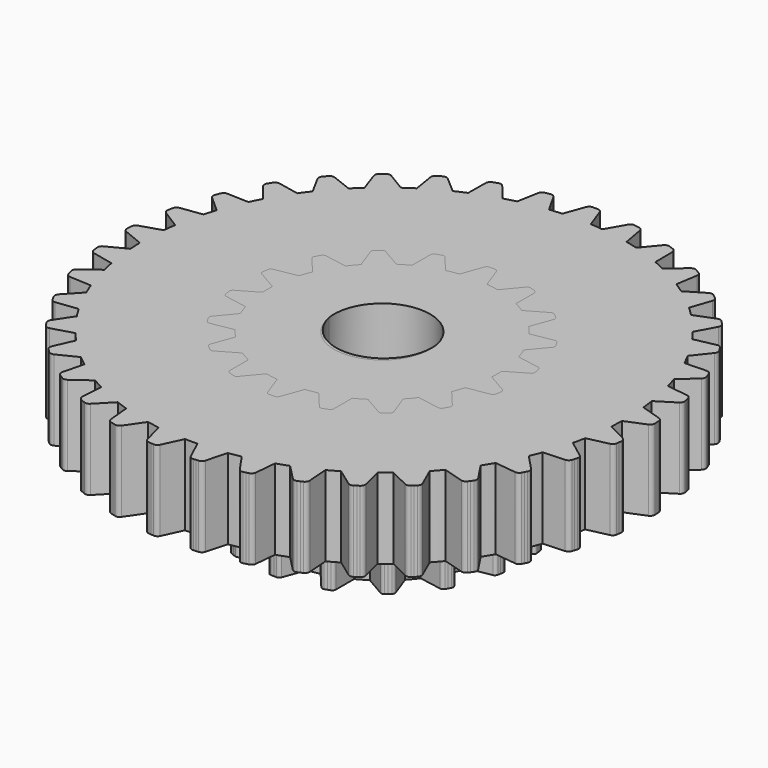
from build123d import *

# Parameters (mm, degrees)
F0_R      = 4.175
F1_DEPTH  = 7
F3_R      = 4.175
F4_DEPTH  = 7
F2_R      = 4.175
F5_DEPTH  = 7
F6_W      = 6
F6_H      = 6
F7_DEPTH  = 3.3
F8_R      = 1.65
F8_R_2    = 0.5
F9_DEPTH  = 0.2
F10_R     = 1.65
F11_DEPTH = 0.7


with BuildPart() as f1:
    # F0 (on Top) → F1 (new body)
    with BuildSketch(Plane.XY):
        with BuildLine():
            ThreePointArc((9.9853543406, -0.5410163509), (9.9963379146, -0.2706072741), (10, 0))
            ThreePointArc((10, 0), (9.9963379146, 0.2706072741), (9.9853543406, 0.5410163509))
            ThreePointArc((9.9853543406, 0.5410163509), (9.8480775301, 1.7364817767), (9.5682022797, 2.9068032501))
            ThreePointArc((9.5682022797, 2.9068032501), (9.3969262079, 3.4202014333), (9.1981253, 3.9235813954))
            ThreePointArc((9.1981253, 3.9235813954), (8.6602540378, 5), (7.9969838122, 6.0040194793))
            ThreePointArc((7.9969838122, 6.0040194793), (7.6604444312, 6.4278760969), (7.3014665983, 6.8329046177))
            ThreePointArc((7.3014665983, 6.8329046177), (6.4278760969, 7.6604444312), (5.461211074, 8.3770623494))
            ThreePointArc((5.461211074, 8.3770623494), (5, 8.6602540378), (4.5241432666, 8.9180787002))
            ThreePointArc((4.5241432666, 8.9180787002), (3.4202014333, 9.3969262079), (2.2667356814, 9.7397078678))
            ThreePointArc((2.2667356814, 9.7397078678), (1.7364817767, 9.8480775301), (1.2011414878, 9.9276008746))
            ThreePointArc((1.2011414878, 9.9276008746), (0.601660724, 9.9818838088), (0, 10))
            ThreePointArc((0, 10), (-0.601660724, 9.9818838088), (-1.2011414878, 9.9276008746))
            ThreePointArc((-1.2011414878, 9.9276008746), (-1.7364817767, 9.8480775301), (-2.2667356814, 9.7397078678))
            ThreePointArc((-2.2667356814, 9.7397078678), (-3.4202014333, 9.3969262079), (-4.5241432666, 8.9180787002))
            ThreePointArc((-4.5241432666, 8.9180787002), (-5, 8.6602540378), (-5.461211074, 8.3770623494))
            ThreePointArc((-5.461211074, 8.3770623494), (-6.4278760969, 7.6604444312), (-7.3014665983, 6.8329046177))
            ThreePointArc((-7.3014665983, 6.8329046177), (-7.6604444312, 6.4278760969), (-7.9969838122, 6.0040194793))
            ThreePointArc((-7.9969838122, 6.0040194793), (-8.6602540378, 5), (-9.1981253, 3.9235813954))
            ThreePointArc((-9.1981253, 3.9235813954), (-9.3969262079, 3.4202014333), (-9.5682022797, 2.9068032501))
            ThreePointArc((-9.5682022797, 2.9068032501), (-9.8480775301, 1.7364817767), (-9.9853543406, 0.5410163509))
            ThreePointArc((-9.9853543406, 0.5410163509), (-10, 0), (-9.9853543406, -0.5410163509))
            ThreePointArc((-9.9853543406, -0.5410163509), (-9.8480775301, -1.7364817767), (-9.5682022797, -2.9068032501))
            ThreePointArc((-9.5682022797, -2.9068032501), (-9.3969262079, -3.4202014333), (-9.1981253, -3.9235813954))
            ThreePointArc((-9.1981253, -3.9235813954), (-8.6602540378, -5), (-7.9969838122, -6.0040194793))
            ThreePointArc((-7.9969838122, -6.0040194793), (-7.6604444312, -6.4278760969), (-7.3014665983, -6.8329046177))
            ThreePointArc((-7.3014665983, -6.8329046177), (-6.4278760969, -7.6604444312), (-5.461211074, -8.3770623494))
            ThreePointArc((-5.461211074, -8.3770623494), (-5, -8.6602540378), (-4.5241432666, -8.9180787002))
            ThreePointArc((-4.5241432666, -8.9180787002), (-3.4202014333, -9.3969262079), (-2.2667356814, -9.7397078678))
            ThreePointArc((-2.2667356814, -9.7397078678), (-1.7364817767, -9.8480775301), (-1.2011414878, -9.9276008746))
            ThreePointArc((-1.2011414878, -9.9276008746), (0, -10), (1.2011414878, -9.9276008746))
            ThreePointArc((1.2011414878, -9.9276008746), (1.7364817767, -9.8480775301), (2.2667356814, -9.7397078678))
            ThreePointArc((2.2667356814, -9.7397078678), (3.4202014333, -9.3969262079), (4.5241432666, -8.9180787002))
            ThreePointArc((4.5241432666, -8.9180787002), (5, -8.6602540378), (5.461211074, -8.3770623494))
            ThreePointArc((5.461211074, -8.3770623494), (6.4278760969, -7.6604444312), (7.3014665983, -6.8329046177))
            ThreePointArc((7.3014665983, -6.8329046177), (7.6604444312, -6.4278760969), (7.9969838122, -6.0040194793))
            ThreePointArc((7.9969838122, -6.0040194793), (8.6602540378, -5), (9.1981253, -3.9235813954))
            ThreePointArc((9.1981253, -3.9235813954), (9.3969262079, -3.4202014333), (9.5682022797, -2.9068032501))
            ThreePointArc((9.5682022797, -2.9068032501), (9.8480775301, -1.7364817767), (9.9853543406, -0.5410163509))
        make_face()
        Circle(F0_R, mode=Mode.SUBTRACT)
        with BuildLine():
            ThreePointArc((9.5682022797, 2.9068032501), (9.8480775301, 1.7364817767), (9.9853543406, 0.5410163509))
            Line((9.9853543406, 0.5410163509), (11.7091989464, 1.5362784981))
            ThreePointArc((11.7091989464, 1.5362784981), (11.8298906667, 1.6667571102), (11.8555661055, 1.8426318708))
            Line((11.8555661055, 1.8426318708), (11.8176930361, 2.083778132))
            Line((11.8176930361, 2.083778132), (11.7708052012, 2.3233348468))
            ThreePointArc((11.7708052012, 2.3233348468), (11.68652547, 2.4798215442), (11.5284860374, 2.5611523338))
            Line((11.5284860374, 2.5611523338), (9.5682022797, 2.9068032501))
        make_face()
        with BuildLine():
            Line((11.7091989464, -1.5362784981), (9.9853543406, -0.5410163509))
            ThreePointArc((9.9853543406, -0.5410163509), (9.8480775301, -1.7364817767), (9.5682022797, -2.9068032501))
            Line((9.5682022797, -2.9068032501), (11.5284860374, -2.5611523338))
            ThreePointArc((11.5284860374, -2.5611523338), (11.68652547, -2.4798215442), (11.7708052012, -2.3233348468))
            Line((11.7708052012, -2.3233348468), (11.8176930361, -2.083778132))
            Line((11.8176930361, -2.083778132), (11.8555661055, -1.8426318708))
            ThreePointArc((11.8555661055, -1.8426318708), (11.8298906667, -1.6667571102), (11.7091989464, -1.5362784981))
        make_face()
        with BuildLine():
            ThreePointArc((7.9969838122, 6.0040194793), (8.6602540378, 5), (9.1981253, 3.9235813954))
            Line((9.1981253, 3.9235813954), (10.4776096532, 5.44841147))
            ThreePointArc((10.4776096532, 5.44841147), (10.5463964585, 5.6123002585), (10.5103707681, 5.7863499905))
            Line((10.5103707681, 5.7863499905), (10.3923048454, 6))
            Line((10.3923048454, 6), (10.266311471, 6.2090730931))
            ThreePointArc((10.266311471, 6.2090730931), (10.1335928268, 6.3272971222), (9.9572675699, 6.3496703956))
            Line((9.9572675699, 6.3496703956), (7.9969838122, 6.0040194793))
        make_face()
        with BuildLine():
            Line((10.4776096532, -5.44841147), (9.1981253, -3.9235813954))
            ThreePointArc((9.1981253, -3.9235813954), (8.6602540378, -5), (7.9969838122, -6.0040194793))
            Line((7.9969838122, -6.0040194793), (9.9572675699, -6.3496703956))
            ThreePointArc((9.9572675699, -6.3496703956), (10.1335928268, -6.3272971222), (10.266311471, -6.2090730931))
            Line((10.266311471, -6.2090730931), (10.3923048454, -6))
            Line((10.3923048454, -6), (10.5103707681, -5.7863499905))
            ThreePointArc((10.5103707681, -5.7863499905), (10.5463964585, -5.6123002585), (10.4776096532, -5.44841147))
        make_face()
        with BuildLine():
            ThreePointArc((5.461211074, 8.3770623494), (6.4278760969, 7.6604444312), (7.3014665983, 6.8329046177))
            Line((7.3014665983, 6.8329046177), (7.9822660027, 8.7033856086))
            ThreePointArc((7.9822660027, 8.7033856086), (7.9908511891, 8.8809171668), (7.8974695994, 9.0321489038))
            Line((7.8974695994, 9.0321489038), (7.7134513162, 9.1925333174))
            Line((7.7134513162, 9.1925333174), (7.5235490627, 9.3459054882))
            ThreePointArc((7.5235490627, 9.3459054882), (7.3583993328, 9.4116072863), (7.1850556798, 9.3723244965))
            Line((7.1850556798, 9.3723244965), (5.461211074, 8.3770623494))
        make_face()
        with BuildLine():
            Line((7.9822660027, -8.7033856086), (7.3014665983, -6.8329046177))
            ThreePointArc((7.3014665983, -6.8329046177), (6.4278760969, -7.6604444312), (5.461211074, -8.3770623494))
            Line((5.461211074, -8.3770623494), (7.1850556798, -9.3723244965))
            ThreePointArc((7.1850556798, -9.3723244965), (7.3583993328, -9.4116072863), (7.5235490627, -9.3459054882))
            Line((7.5235490627, -9.3459054882), (7.7134513162, -9.1925333174))
            Line((7.7134513162, -9.1925333174), (7.8974695994, -9.0321489038))
            ThreePointArc((7.8974695994, -9.0321489038), (7.9908511891, -8.8809171668), (7.9822660027, -8.7033856086))
        make_face()
        with BuildLine():
            ThreePointArc((2.2667356814, 9.7397078678), (3.4202014333, 9.3969262079), (4.5241432666, 8.9180787002))
            Line((4.5241432666, 8.9180787002), (4.5241432666, 10.9086029946))
            ThreePointArc((4.5241432666, 10.9086029946), (4.471491334, 11.0783643965), (4.3320170428, 11.1885373591))
            Line((4.3320170428, 11.1885373591), (4.1042417199, 11.2763114494))
            Line((4.1042417199, 11.2763114494), (3.8733356018, 11.3554837506))
            ThreePointArc((3.8733356018, 11.3554837506), (3.6956742808, 11.3607387111), (3.5462200347, 11.2645379424))
            Line((3.5462200347, 11.2645379424), (2.2667356814, 9.7397078678))
        make_face()
        with BuildLine():
            Line((4.5241432666, -10.9086029946), (4.5241432666, -8.9180787002))
            ThreePointArc((4.5241432666, -8.9180787002), (3.4202014333, -9.3969262079), (2.2667356814, -9.7397078678))
            Line((2.2667356814, -9.7397078678), (3.5462200347, -11.2645379424))
            ThreePointArc((3.5462200347, -11.2645379424), (3.6956742808, -11.3607387111), (3.8733356018, -11.3554837506))
            Line((3.8733356018, -11.3554837506), (4.1042417199, -11.2763114494))
            Line((4.1042417199, -11.2763114494), (4.3320170428, -11.1885373591))
            ThreePointArc((4.3320170428, -11.1885373591), (4.471491334, -11.0783643965), (4.5241432666, -10.9086029946))
        make_face()
        with BuildLine():
            ThreePointArc((0, 10), (0.601660724, 9.9818838088), (1.2011414878, 9.9276008746))
            Line((1.2011414878, 9.9276008746), (0.5203420833, 11.7980818656))
            ThreePointArc((0.5203420833, 11.7980818656), (0.4128036317, 11.9395973807), (0.2440592971, 11.9954230836))
            Line((0.2440592971, 11.9954230836), (0, 12))
            Line((0, 12), (0, 10))
        make_face()
        with BuildLine():
            Line((0.5203420833, -11.7980818656), (1.2011414878, -9.9276008746))
            ThreePointArc((1.2011414878, -9.9276008746), (0, -10), (-1.2011414878, -9.9276008746))
            Line((-1.2011414878, -9.9276008746), (-0.5203420833, -11.7980818656))
            ThreePointArc((-0.5203420833, -11.7980818656), (-0.4128036317, -11.9395973807), (-0.2440592971, -11.9954230836))
            Line((-0.2440592971, -11.9954230836), (0, -12))
            Line((0, -12), (0.2440592971, -11.9954230836))
            ThreePointArc((0.2440592971, -11.9954230836), (0.4128036317, -11.9395973807), (0.5203420833, -11.7980818656))
        make_face()
        with BuildLine():
            ThreePointArc((-1.2011414878, 9.9276008746), (-0.601660724, 9.9818838088), (0, 10))
            Line((0, 10), (0, 12))
            Line((0, 12), (-0.2440592971, 11.9954230836))
            ThreePointArc((-0.2440592971, 11.9954230836), (-0.4128036317, 11.9395973807), (-0.5203420833, 11.7980818656))
            Line((-0.5203420833, 11.7980818656), (-1.2011414878, 9.9276008746))
        make_face()
        with BuildLine():
            Line((-3.5462200347, -11.2645379424), (-2.2667356814, -9.7397078678))
            ThreePointArc((-2.2667356814, -9.7397078678), (-3.4202014333, -9.3969262079), (-4.5241432666, -8.9180787002))
            Line((-4.5241432666, -8.9180787002), (-4.5241432666, -10.9086029946))
            ThreePointArc((-4.5241432666, -10.9086029946), (-4.471491334, -11.0783643965), (-4.3320170428, -11.1885373591))
            Line((-4.3320170428, -11.1885373591), (-4.1042417199, -11.2763114494))
            Line((-4.1042417199, -11.2763114494), (-3.8733356018, -11.3554837506))
            ThreePointArc((-3.8733356018, -11.3554837506), (-3.6956742808, -11.3607387111), (-3.5462200347, -11.2645379424))
        make_face()
        with BuildLine():
            ThreePointArc((-4.5241432666, 8.9180787002), (-3.4202014333, 9.3969262079), (-2.2667356814, 9.7397078678))
            Line((-2.2667356814, 9.7397078678), (-3.5462200347, 11.2645379424))
            ThreePointArc((-3.5462200347, 11.2645379424), (-3.6956742808, 11.3607387111), (-3.8733356018, 11.3554837506))
            Line((-3.8733356018, 11.3554837506), (-4.1042417199, 11.2763114494))
            Line((-4.1042417199, 11.2763114494), (-4.3320170428, 11.1885373591))
            ThreePointArc((-4.3320170428, 11.1885373591), (-4.471491334, 11.0783643965), (-4.5241432666, 10.9086029946))
            Line((-4.5241432666, 10.9086029946), (-4.5241432666, 8.9180787002))
        make_face()
        with BuildLine():
            Line((-7.1850556798, -9.3723244965), (-5.461211074, -8.3770623494))
            ThreePointArc((-5.461211074, -8.3770623494), (-6.4278760969, -7.6604444312), (-7.3014665983, -6.8329046177))
            Line((-7.3014665983, -6.8329046177), (-7.9822660027, -8.7033856086))
            ThreePointArc((-7.9822660027, -8.7033856086), (-7.9908511891, -8.8809171668), (-7.8974695994, -9.0321489038))
            Line((-7.8974695994, -9.0321489038), (-7.7134513162, -9.1925333174))
            Line((-7.7134513162, -9.1925333174), (-7.5235490627, -9.3459054882))
            ThreePointArc((-7.5235490627, -9.3459054882), (-7.3583993328, -9.4116072863), (-7.1850556798, -9.3723244965))
        make_face()
        with BuildLine():
            ThreePointArc((-7.3014665983, 6.8329046177), (-6.4278760969, 7.6604444312), (-5.461211074, 8.3770623494))
            Line((-5.461211074, 8.3770623494), (-7.1850556798, 9.3723244965))
            ThreePointArc((-7.1850556798, 9.3723244965), (-7.3583993328, 9.4116072863), (-7.5235490627, 9.3459054882))
            Line((-7.5235490627, 9.3459054882), (-7.7134513162, 9.1925333174))
            Line((-7.7134513162, 9.1925333174), (-7.8974695994, 9.0321489038))
            ThreePointArc((-7.8974695994, 9.0321489038), (-7.9908511891, 8.8809171668), (-7.9822660027, 8.7033856086))
            Line((-7.9822660027, 8.7033856086), (-7.3014665983, 6.8329046177))
        make_face()
        with BuildLine():
            Line((-9.9572675699, -6.3496703956), (-7.9969838122, -6.0040194793))
            ThreePointArc((-7.9969838122, -6.0040194793), (-8.6602540378, -5), (-9.1981253, -3.9235813954))
            Line((-9.1981253, -3.9235813954), (-10.4776096532, -5.44841147))
            ThreePointArc((-10.4776096532, -5.44841147), (-10.5463964585, -5.6123002585), (-10.5103707681, -5.7863499905))
            Line((-10.5103707681, -5.7863499905), (-10.3923048454, -6))
            Line((-10.3923048454, -6), (-10.266311471, -6.2090730931))
            ThreePointArc((-10.266311471, -6.2090730931), (-10.1335928268, -6.3272971222), (-9.9572675699, -6.3496703956))
        make_face()
        with BuildLine():
            ThreePointArc((-9.1981253, 3.9235813954), (-8.6602540378, 5), (-7.9969838122, 6.0040194793))
            Line((-7.9969838122, 6.0040194793), (-9.9572675699, 6.3496703956))
            ThreePointArc((-9.9572675699, 6.3496703956), (-10.1335928268, 6.3272971222), (-10.266311471, 6.2090730931))
            Line((-10.266311471, 6.2090730931), (-10.3923048454, 6))
            Line((-10.3923048454, 6), (-10.5103707681, 5.7863499905))
            ThreePointArc((-10.5103707681, 5.7863499905), (-10.5463964585, 5.6123002585), (-10.4776096532, 5.44841147))
            Line((-10.4776096532, 5.44841147), (-9.1981253, 3.9235813954))
        make_face()
        with BuildLine():
            Line((-11.5284860374, -2.5611523338), (-9.5682022797, -2.9068032501))
            ThreePointArc((-9.5682022797, -2.9068032501), (-9.8480775301, -1.7364817767), (-9.9853543406, -0.5410163509))
            Line((-9.9853543406, -0.5410163509), (-11.7091989464, -1.5362784981))
            ThreePointArc((-11.7091989464, -1.5362784981), (-11.8298906667, -1.6667571102), (-11.8555661055, -1.8426318708))
            Line((-11.8555661055, -1.8426318708), (-11.8176930361, -2.083778132))
            Line((-11.8176930361, -2.083778132), (-11.7708052012, -2.3233348468))
            ThreePointArc((-11.7708052012, -2.3233348468), (-11.68652547, -2.4798215442), (-11.5284860374, -2.5611523338))
        make_face()
        with BuildLine():
            ThreePointArc((-9.9853543406, 0.5410163509), (-9.8480775301, 1.7364817767), (-9.5682022797, 2.9068032501))
            Line((-9.5682022797, 2.9068032501), (-11.5284860374, 2.5611523338))
            ThreePointArc((-11.5284860374, 2.5611523338), (-11.68652547, 2.4798215442), (-11.7708052012, 2.3233348468))
            Line((-11.7708052012, 2.3233348468), (-11.8176930361, 2.083778132))
            Line((-11.8176930361, 2.083778132), (-11.8555661055, 1.8426318708))
            ThreePointArc((-11.8555661055, 1.8426318708), (-11.8298906667, 1.6667571102), (-11.7091989464, 1.5362784981))
            Line((-11.7091989464, 1.5362784981), (-9.9853543406, 0.5410163509))
        make_face()
    extrude(amount=F1_DEPTH)

    # F2 (on face) → F5 (join)
    with BuildSketch(Plane.XY.offset(7)):
        with BuildLine():
            ThreePointArc((20.9971088354, -0.3484545248), (20.9992771964, -0.1742332594), (21, 0))
            ThreePointArc((21, 0), (20.9729614688, 1.0653108598), (20.8919155021, 2.1278784395))
            ThreePointArc((20.8919155021, 2.1278784395), (20.8299091404, 2.6673742147), (20.75397364, 3.2050862938))
            ThreePointArc((20.75397364, 3.2050862938), (20.5286600179, 4.4242646699), (20.2317911147, 5.6280217032))
            ThreePointArc((20.2317911147, 5.6280217032), (20.0795014295, 6.1492781968), (19.9137844096, 6.6664226153))
            ThreePointArc((19.9137844096, 6.6664226153), (19.4856695732, 7.8299860334), (18.9896349328, 8.9662570294))
            ThreePointArc((18.9896349328, 8.9662570294), (18.7514430211, 9.4542786412), (18.5007118588, 9.9359780957))
            ThreePointArc((18.5007118588, 9.9359780957), (17.8821118924, 11.0104529547), (17.2011815283, 12.0465494658))
            ThreePointArc((17.2011815283, 12.0465494658), (16.8839397377, 12.4872967024), (16.5554075119, 12.9196935767))
            ThreePointArc((16.5554075119, 12.9196935767), (15.7641184103, 13.8741691912), (14.9178814493, 14.780284607))
            ThreePointArc((14.9178814493, 14.780284607), (14.5307162485, 15.161077973), (14.1338342332, 15.5317329963))
            ThreePointArc((14.1338342332, 15.5317329963), (13.1926199432, 16.3387508407), (12.2054210819, 17.0888178705))
            ThreePointArc((12.2054210819, 17.0888178705), (11.7594705089, 17.3987026341), (11.3056562771, 17.6969527361))
            ThreePointArc((11.3056562771, 17.6969527361), (10.2415938201, 18.3332963764), (9.1418329724, 18.9057369575))
            ThreePointArc((9.1418329724, 18.9057369575), (8.6499262131, 19.1357982982), (8.152235174, 19.3530633665))
            ThreePointArc((8.152235174, 19.3530633665), (6.9959356896, 19.8004263547), (5.8152509727, 20.1787724137))
            ThreePointArc((5.8152509727, 20.1787724137), (5.2915392891, 20.3223918856), (4.7642891078, 20.4524215998))
            ThreePointArc((4.7642891078, 20.4524215998), (3.5490172268, 20.6979341173), (2.3213747904, 20.871301327))
            ThreePointArc((2.3213747904, 20.871301327), (1.780924414, 20.9243472594), (1.2392831182, 20.9634009014))
            ThreePointArc((1.2392831182, 20.9634009014), (0, 21), (-1.2392831182, 20.9634009014))
            ThreePointArc((-1.2392831182, 20.9634009014), (-1.780924414, 20.9243472594), (-2.3213747904, 20.871301327))
            ThreePointArc((-2.3213747904, 20.871301327), (-3.5490172268, 20.6979341173), (-4.7642891078, 20.4524215998))
            ThreePointArc((-4.7642891078, 20.4524215998), (-5.2915392891, 20.3223918856), (-5.8152509727, 20.1787724137))
            ThreePointArc((-5.8152509727, 20.1787724137), (-6.9959356896, 19.8004263547), (-8.152235174, 19.3530633665))
            ThreePointArc((-8.152235174, 19.3530633665), (-8.6499262131, 19.1357982982), (-9.1418329724, 18.9057369575))
            ThreePointArc((-9.1418329724, 18.9057369575), (-10.2415938201, 18.3332963764), (-11.3056562771, 17.6969527361))
            ThreePointArc((-11.3056562771, 17.6969527361), (-11.7594705089, 17.3987026341), (-12.2054210819, 17.0888178705))
            ThreePointArc((-12.2054210819, 17.0888178705), (-13.1926199432, 16.3387508407), (-14.1338342332, 15.5317329963))
            ThreePointArc((-14.1338342332, 15.5317329963), (-14.5307162485, 15.161077973), (-14.9178814493, 14.780284607))
            ThreePointArc((-14.9178814493, 14.780284607), (-15.7641184103, 13.8741691912), (-16.5554075119, 12.9196935767))
            ThreePointArc((-16.5554075119, 12.9196935767), (-16.8839397377, 12.4872967024), (-17.2011815283, 12.0465494658))
            ThreePointArc((-17.2011815283, 12.0465494658), (-17.8821118924, 11.0104529547), (-18.5007118588, 9.9359780957))
            ThreePointArc((-18.5007118588, 9.9359780957), (-18.7514430211, 9.4542786412), (-18.9896349328, 8.9662570294))
            ThreePointArc((-18.9896349328, 8.9662570294), (-19.4856695732, 7.8299860334), (-19.9137844096, 6.6664226153))
            ThreePointArc((-19.9137844096, 6.6664226153), (-20.0795014295, 6.1492781968), (-20.2317911147, 5.6280217032))
            ThreePointArc((-20.2317911147, 5.6280217032), (-20.5286600179, 4.4242646699), (-20.75397364, 3.2050862938))
            ThreePointArc((-20.75397364, 3.2050862938), (-20.8299091404, 2.6673742147), (-20.8919155021, 2.1278784395))
            ThreePointArc((-20.8919155021, 2.1278784395), (-20.9810782903, 0.8912652671), (-20.9971088354, -0.3484545248))
            ThreePointArc((-20.9971088354, -0.3484545248), (-20.9810782903, -0.8912652671), (-20.9510175183, -1.4334800127))
            ThreePointArc((-20.9510175183, -1.4334800127), (-20.8299091404, -2.6673742147), (-20.6361954389, -3.8919709413))
            ThreePointArc((-20.6361954389, -3.8919709413), (-20.5286600179, -4.4242646699), (-20.407396906, -4.9535998548))
            ThreePointArc((-20.407396906, -4.9535998548), (-20.0795014295, -6.1492781968), (-19.6816162719, -7.3235224398))
            ThreePointArc((-19.6816162719, -7.3235224398), (-19.4856695732, -7.8299860334), (-19.2766926403, -8.3312136482))
            ThreePointArc((-19.2766926403, -8.3312136482), (-18.7514430211, -9.4542786412), (-18.1608328389, -10.5443895317))
            ThreePointArc((-18.1608328389, -10.5443895317), (-17.8821118924, -11.0104529547), (-17.5914330244, -11.4691535934))
            ThreePointArc((-17.5914330244, -11.4691535934), (-16.8839397377, -12.4872967024), (-16.1175953106, -13.4619137349))
            ThreePointArc((-16.1175953106, -13.4619137349), (-15.7641184103, -13.8741691912), (-15.4000999089, -14.2771468717))
            ThreePointArc((-15.4000999089, -14.2771468717), (-14.5307162485, -15.161077973), (-13.6106839104, -15.9921631899))
            ThreePointArc((-13.6106839104, -15.9921631899), (-13.1926199432, -16.3387508407), (-12.765733958, -16.6744126287))
            ThreePointArc((-12.765733958, -16.6744126287), (-11.7594705089, -17.3987026341), (-10.7122179149, -18.0623472268))
            ThreePointArc((-10.7122179149, -18.0623472268), (-10.2415938201, -18.3332963764), (-9.7641210837, -18.5919858935))
            ThreePointArc((-9.7641210837, -18.5919858935), (-8.6499262131, -19.1357982982), (-7.5055809138, -19.6129104201))
            ThreePointArc((-7.5055809138, -19.6129104201), (-6.9959356896, -19.8004263547), (-6.4816122232, -19.9747015744))
            ThreePointArc((-6.4816122232, -19.9747015744), (-5.2915392891, -20.3223918856), (-4.0830220152, -20.5992458897))
            ThreePointArc((-4.0830220152, -20.5992458897), (-3.5490172268, -20.6979341173), (-3.0126391801, -20.7827814589))
            ThreePointArc((-3.0126391801, -20.7827814589), (-1.780924414, -20.9243472594), (-0.5430020071, -20.99297856))
            ThreePointArc((-0.5430020071, -20.99297856), (0, -21), (0.5430020071, -20.99297856))
            ThreePointArc((0.5430020071, -20.99297856), (1.780924414, -20.9243472594), (3.0126391801, -20.7827814589))
            ThreePointArc((3.0126391801, -20.7827814589), (3.5490172268, -20.6979341173), (4.0830220152, -20.5992458897))
            ThreePointArc((4.0830220152, -20.5992458897), (5.2915392891, -20.3223918856), (6.4816122232, -19.9747015744))
            ThreePointArc((6.4816122232, -19.9747015744), (6.9959356896, -19.8004263547), (7.5055809138, -19.6129104201))
            ThreePointArc((7.5055809138, -19.6129104201), (8.6499262131, -19.1357982982), (9.7641210837, -18.5919858935))
            ThreePointArc((9.7641210837, -18.5919858935), (10.2415938201, -18.3332963764), (10.7122179149, -18.0623472268))
            ThreePointArc((10.7122179149, -18.0623472268), (11.7594705089, -17.3987026341), (12.765733958, -16.6744126287))
            ThreePointArc((12.765733958, -16.6744126287), (13.1926199432, -16.3387508407), (13.6106839104, -15.9921631899))
            ThreePointArc((13.6106839104, -15.9921631899), (14.5307162485, -15.161077973), (15.4000999089, -14.2771468717))
            ThreePointArc((15.4000999089, -14.2771468717), (15.7641184103, -13.8741691912), (16.1175953106, -13.4619137349))
            ThreePointArc((16.1175953106, -13.4619137349), (16.8839397377, -12.4872967024), (17.5914330244, -11.4691535934))
            ThreePointArc((17.5914330244, -11.4691535934), (17.8821118924, -11.0104529547), (18.1608328389, -10.5443895317))
            ThreePointArc((18.1608328389, -10.5443895317), (18.7514430211, -9.4542786412), (19.2766926403, -8.3312136482))
            ThreePointArc((19.2766926403, -8.3312136482), (19.4856695732, -7.8299860334), (19.6816162719, -7.3235224398))
            ThreePointArc((19.6816162719, -7.3235224398), (20.0795014295, -6.1492781968), (20.407396906, -4.9535998548))
            ThreePointArc((20.407396906, -4.9535998548), (20.5286600179, -4.4242646699), (20.6361954389, -3.8919709413))
            ThreePointArc((20.6361954389, -3.8919709413), (20.8299091404, -2.6673742147), (20.9510175183, -1.4334800127))
            ThreePointArc((20.9510175183, -1.4334800127), (20.9810782903, -0.8912652671), (20.9971088354, -0.3484545248))
        make_face()
        Circle(F2_R, mode=Mode.SUBTRACT)
        with BuildLine():
            ThreePointArc((20.8919155021, 2.1278784395), (20.9729614688, 1.0653108598), (21, 0))
            ThreePointArc((21, 0), (20.9992771964, -0.1742332594), (20.9971088354, -0.3484545248))
            Line((20.9971088354, -0.3484545248), (22.7391606338, 0.370721297))
            ThreePointArc((22.7391606338, 0.370721297), (22.9224507952, 0.5233068025), (22.9863236836, 0.7530846819))
            Line((22.9863236836, 0.7530846819), (22.9792762227, 0.9761476735))
            Line((22.9792762227, 0.9761476735), (22.9673812318, 1.1990047446))
            ThreePointArc((22.9673812318, 1.1990047446), (22.8842519207, 1.4225380472), (22.6886819094, 1.55902977))
            Line((22.6886819094, 1.55902977), (20.8919155021, 2.1278784395))
        make_face()
        with BuildLine():
            ThreePointArc((20.2317911147, 5.6280217032), (20.5286600179, 4.4242646699), (20.75397364, 3.2050862938))
            Line((20.75397364, 3.2050862938), (22.3494263053, 4.2083256092))
            ThreePointArc((22.3494263053, 4.2083256092), (22.504292929, 4.3896924987), (22.5284144139, 4.626959803))
            Line((22.5284144139, 4.626959803), (22.4837704958, 4.8456232099))
            Line((22.4837704958, 4.8456232099), (22.4343835757, 5.0632644217))
            ThreePointArc((22.4343835757, 5.0632644217), (22.3146726925, 5.2695334794), (22.0988485646, 5.3710104008))
            Line((22.0988485646, 5.3710104008), (20.2317911147, 5.6280217032))
        make_face()
        with BuildLine():
            Line((22.6258031847, -2.2978013086), (20.9510175183, -1.4334800127))
            ThreePointArc((20.9510175183, -1.4334800127), (20.8299091404, -2.6673742147), (20.6361954389, -3.8919709413))
            Line((20.6361954389, -3.8919709413), (22.4747307119, -3.4775479919))
            ThreePointArc((22.4747307119, -3.4775479919), (22.6811714868, -3.3581334776), (22.782958272, -3.1424553144))
            Line((22.782958272, -3.1424553144), (22.813710011, -2.9214098542))
            Line((22.813710011, -2.9214098542), (22.8396491465, -2.699748116))
            ThreePointArc((22.8396491465, -2.699748116), (22.7954928864, -2.4653812147), (22.6258031847, -2.2978013086))
        make_face()
        with BuildLine():
            ThreePointArc((18.9896349328, 8.9662570294), (19.4856695732, 7.8299860334), (19.9137844096, 6.6664226153))
            Line((19.9137844096, 6.6664226153), (21.3167396735, 7.9248640556))
            ThreePointArc((21.3167396735, 7.9248640556), (21.4387275287, 8.129794734), (21.422403679, 8.3677257149))
            Line((21.422403679, 8.3677257149), (21.3414476278, 8.5756989889))
            Line((21.3414476278, 8.5756989889), (21.2559895503, 8.7818632))
            ThreePointArc((21.2559895503, 8.7818632), (21.1031409592, 8.9649340277), (20.873271582, 9.0284768412))
            Line((20.873271582, 9.0284768412), (18.9896349328, 8.9662570294))
        make_face()
        with BuildLine():
            Line((21.9120212972, -6.0885288273), (20.407396906, -4.9535998548))
            ThreePointArc((20.407396906, -4.9535998548), (20.0795014295, -6.1492781968), (19.6816162719, -7.3235224398))
            Line((19.6816162719, -7.3235224398), (21.5637437071, -7.2257745566))
            ThreePointArc((21.5637437071, -7.2257745566), (21.7873961702, -7.1429663718), (21.9241686317, -6.9475925927))
            Line((21.9241686317, -6.9475925927), (21.991834899, -6.7349237394))
            Line((21.991834899, -6.7349237394), (22.0548619393, -6.5208341387))
            ThreePointArc((22.0548619393, -6.5208341387), (22.0509490253, -6.2823759477), (21.9120212972, -6.0885288273))
        make_face()
        with BuildLine():
            ThreePointArc((17.2011815283, 12.0465494658), (17.8821118924, 11.0104529547), (18.5007118588, 9.9359780957))
            Line((18.5007118588, 9.9359780957), (19.6708092526, 11.413418592))
            ThreePointArc((19.6708092526, 11.413418592), (19.7564089708, 11.6360175767), (19.7001093938, 11.8677673931))
            Line((19.7001093938, 11.8677673931), (19.5851701679, 12.0590675218))
            Line((19.5851701679, 12.0590675218), (19.4660994062, 12.2478237632))
            ThreePointArc((19.4660994062, 12.2478237632), (19.2845102829, 12.4024297464), (19.0472085798, 12.4262104411))
            Line((19.0472085798, 12.4262104411), (17.2011815283, 12.0465494658))
        make_face()
        with BuildLine():
            Line((20.567870452, -9.7041004569), (19.2766926403, -8.3312136482))
            ThreePointArc((19.2766926403, -8.3312136482), (18.7514430211, -9.4542786412), (18.1608328389, -10.5443895317))
            Line((18.1608328389, -10.5443895317), (20.0324070568, -10.7661287433))
            ThreePointArc((20.0324070568, -10.7661287433), (20.2668371341, -10.7223091285), (20.4346605771, -10.5528602817))
            Line((20.4346605771, -10.5528602817), (20.5372947374, -10.3546861308))
            Line((20.5372947374, -10.3546861308), (20.6355965093, -10.1543276356))
            ThreePointArc((20.6355965093, -10.1543276356), (20.6720395089, -9.918638163), (20.567870452, -9.7041004569))
        make_face()
        with BuildLine():
            ThreePointArc((14.9178814493, 14.780284607), (15.7641184103, 13.8741691912), (16.5554075119, 12.9196935767))
            Line((16.5554075119, 12.9196935767), (17.458985464, 14.5736298558))
            ThreePointArc((17.458985464, 14.5736298558), (17.5057344972, 14.8074933794), (17.4110788294, 15.0263950109))
            Line((17.4110788294, 15.0263950109), (17.2654630208, 15.195518638))
            Line((17.2654630208, 15.195518638), (17.116205024, 15.3614367362))
            ThreePointArc((17.116205024, 15.3614367362), (16.911099357, 15.4831301423), (16.6731920659, 15.4664645909))
            Line((16.6731920659, 15.4664645909), (14.9178814493, 14.780284607))
        make_face()
        with BuildLine():
            Line((18.6320194218, -13.0405027846), (17.5914330244, -11.4691535934))
            ThreePointArc((17.5914330244, -11.4691535934), (16.8839397377, -12.4872967024), (16.1175953106, -13.4619137349))
            Line((16.1175953106, -13.4619137349), (17.9247745285, -13.9967610079))
            ThreePointArc((17.9247745285, -13.9967610079), (18.1632380933, -13.9931905737), (18.357284543, -13.8545413938))
            Line((18.357284543, -13.8545413938), (18.4919339984, -13.676563055))
            Line((18.4919339984, -13.676563055), (18.6226825388, -13.4956996145))
            ThreePointArc((18.6226825388, -13.4956996145), (18.6984330533, -13.2695592171), (18.6320194218, -13.0405027846))
        make_face()
        with BuildLine():
            ThreePointArc((12.2054210819, 17.0888178705), (13.1926199432, 16.3387508407), (14.1338342332, 15.5317329963))
            Line((14.1338342332, 15.5317329963), (14.7448984512, 17.3145843228))
            ThreePointArc((14.7448984512, 17.3145843228), (14.7514519147, 17.5529845574), (14.6211632272, 17.7527406028))
            Line((14.6211632272, 17.7527406028), (14.4490599378, 17.8948223493))
            Line((14.4490599378, 17.8948223493), (14.2739085867, 18.0331291429))
            ThreePointArc((14.2739085867, 18.0331291429), (14.0511868925, 18.1184090741), (13.8195181731, 18.0617767141))
            Line((13.8195181731, 18.0617767141), (12.2054210819, 17.0888178705))
        make_face()
        with BuildLine():
            Line((16.160159116, -16.00175359), (15.4000999089, -14.2771468717))
            ThreePointArc((15.4000999089, -14.2771468717), (14.5307162485, -15.161077973), (13.6106839104, -15.9921631899))
            Line((13.6106839104, -15.9921631899), (15.3014788725, -16.8247319421))
            ThreePointArc((15.3014788725, -16.8247319421), (15.5371157623, -16.8615134035), (15.7518028556, -16.757652575))
            Line((15.7518028556, -16.757652575), (15.9145939865, -16.604990161))
            Line((15.9145939865, -16.604990161), (16.0740278979, -16.4488248869))
            ThreePointArc((16.0740278979, -16.4488248869), (16.1869067229, -16.2387392125), (16.160159116, -16.00175359))
        make_face()
        with BuildLine():
            ThreePointArc((9.1418329724, 18.9057369575), (10.2415938201, 18.3332963764), (11.3056562771, 17.6969527361))
            Line((11.3056562771, 17.6969527361), (11.6066275559, 19.5574297234))
            ThreePointArc((11.6066275559, 19.5574297234), (11.5727969186, 19.7935083284), (11.4106233797, 19.9683721698))
            Line((11.4106233797, 19.9683721698), (11.2169837077, 20.0793246027))
            Line((11.2169837077, 20.0793246027), (11.0209777878, 20.1860412569))
            ThreePointArc((11.0209777878, 20.1860412569), (10.7870473641, 20.232454365), (10.5682819036, 20.1374844063))
            Line((10.5682819036, 20.1374844063), (9.1418329724, 18.9057369575))
        make_face()
        with BuildLine():
            Line((13.2234004552, -18.5026630789), (12.765733958, -16.6744126287))
            ThreePointArc((12.765733958, -16.6744126287), (11.7594705089, -17.3987026341), (10.7122179149, -18.0623472268))
            Line((10.7122179149, -18.0623472268), (12.2379875286, -19.1686859711))
            ThreePointArc((12.2379875286, -19.1686859711), (12.4640188992, -19.2447611923), (12.6931704793, -19.1786766021))
            Line((12.6931704793, -19.1786766021), (12.8794200812, -19.0557219326))
            Line((12.8794200812, -19.0557219326), (13.0629527404, -18.9287474157))
            ThreePointArc((13.0629527404, -18.9287474157), (13.2097125575, -18.7407602464), (13.2234004552, -18.5026630789))
        make_face()
        with BuildLine():
            ThreePointArc((5.8152509727, 20.1787724137), (6.9959356896, 19.8004263547), (8.152235174, 19.3530633665))
            Line((8.152235174, 19.3530633665), (8.1344551179, 21.237643479))
            ThreePointArc((8.1344551179, 21.237643479), (8.0612136256, 21.4646089027), (7.8718206728, 21.6095500259))
            Line((7.8718206728, 21.6095500259), (7.6622152791, 21.6861812456))
            Line((7.6622152791, 21.6861812456), (7.4509935238, 21.7582377166))
            ThreePointArc((7.4509935238, 21.7582377166), (7.2125841229, 21.7644487809), (7.0130154053, 21.6338733363))
            Line((7.0130154053, 21.6338733363), (5.8152509727, 20.1787724137))
        make_face()
        with BuildLine():
            Line((9.9062286391, -20.4712846387), (9.7641210837, -18.5919858935))
            ThreePointArc((9.7641210837, -18.5919858935), (8.6499262131, -19.1357982982), (7.5055809138, -19.6129104201))
            Line((7.5055809138, -19.6129104201), (8.8224315653, -20.961191805))
            ThreePointArc((8.8224315653, -20.961191805), (9.0323549055, -21.0743722404), (9.2693786987, -21.0479650219))
            Line((9.2693786987, -21.0479650219), (9.4737287096, -20.9582552789))
            Line((9.4737287096, -20.9582552789), (9.6760802161, -20.8641243448))
            ThreePointArc((9.6760802161, -20.8641243448), (9.8524990127, -20.7036437293), (9.9062286391, -20.4712846387))
        make_face()
        with BuildLine():
            ThreePointArc((2.3213747904, 20.871301327), (3.5490172268, 20.6979341173), (4.7642891078, 20.4524215998))
            Line((4.7642891078, 20.4524215998), (4.4282692166, 22.306888899))
            ThreePointArc((4.4282692166, 22.306888899), (4.3177238937, 22.5182117595), (4.1065600174, 22.6290604721))
            Line((4.1065600174, 22.6290604721), (3.8870188674, 22.669165938))
            Line((3.8870188674, 22.669165938), (3.666657742, 22.7044892924))
            ThreePointArc((3.666657742, 22.7044892924), (3.4306279684, 22.6703196318), (3.2559972224, 22.5078951192))
            Line((3.2559972224, 22.5078951192), (2.3213747904, 20.871301327))
        make_face()
        with BuildLine():
            Line((6.3040726612, -21.8509846115), (6.4816122232, -19.9747015744))
            ThreePointArc((6.4816122232, -19.9747015744), (5.2915392891, -20.3223918856), (4.0830220152, -20.5992458897))
            Line((4.0830220152, -20.5992458897), (5.1530703087, -22.1506823146))
            ThreePointArc((5.1530703087, -22.1506823146), (5.3408465064, -22.2977119692), (5.5789237697, -22.31174181))
            Line((5.5789237697, -22.31174181), (5.7954954119, -22.2578577795))
            Line((5.7954954119, -22.2578577795), (6.0108444812, -22.1992784038))
            ThreePointArc((6.0108444812, -22.1992784038), (6.2118470097, -22.0709210772), (6.3040726612, -21.8509846115))
        make_face()
        with BuildLine():
            ThreePointArc((-1.2392831182, 20.9634009014), (0, 21), (1.2392831182, 20.9634009014))
            Line((1.2392831182, 20.9634009014), (0.5946900724, 22.7344057394))
            ThreePointArc((0.5946900724, 22.7344057394), (0.4500211066, 22.9240066627), (0.223161107, 22.9975740491))
            Line((0.223161107, 22.9975740491), (0, 23))
            Line((0, 23), (-0.223161107, 22.9975740491))
            ThreePointArc((-0.223161107, 22.9975740491), (-0.4500211066, 22.9240066627), (-0.5946900724, 22.7344057394))
            Line((-0.5946900724, 22.7344057394), (-1.2392831182, 20.9634009014))
        make_face()
        with BuildLine():
            Line((2.5205599907, -22.6020715409), (3.0126391801, -20.7827814589))
            ThreePointArc((3.0126391801, -20.7827814589), (1.780924414, -20.9243472594), (0.5430020071, -20.99297856))
            Line((0.5430020071, -20.99297856), (1.3354646016, -22.7029380237))
            ThreePointArc((1.3354646016, -22.7029380237), (1.4956916773, -22.879587122), (1.7279733613, -22.9336504091))
            Line((1.7279733613, -22.9336504091), (1.9505362629, -22.9171422365))
            Line((1.9505362629, -22.9171422365), (2.1726876945, -22.8957996411))
            ThreePointArc((2.1726876945, -22.8957996411), (2.3924914781, -22.80325821), (2.5205599907, -22.6020715409))
        make_face()
        with BuildLine():
            ThreePointArc((-4.7642891078, 20.4524215998), (-3.5490172268, 20.6979341173), (-2.3213747904, 20.871301327))
            Line((-2.3213747904, 20.871301327), (-3.2559972224, 22.5078951192))
            ThreePointArc((-3.2559972224, 22.5078951192), (-3.4306279684, 22.6703196318), (-3.666657742, 22.7044892924))
            Line((-3.666657742, 22.7044892924), (-3.8870188674, 22.669165938))
            Line((-3.8870188674, 22.669165938), (-4.1065600174, 22.6290604721))
            ThreePointArc((-4.1065600174, 22.6290604721), (-4.3177238937, 22.5182117595), (-4.4282692166, 22.306888899))
            Line((-4.4282692166, 22.306888899), (-4.7642891078, 20.4524215998))
        make_face()
        with BuildLine():
            Line((-1.3354646016, -22.7029380237), (-0.5430020071, -20.99297856))
            ThreePointArc((-0.5430020071, -20.99297856), (-1.780924414, -20.9243472594), (-3.0126391801, -20.7827814589))
            Line((-3.0126391801, -20.7827814589), (-2.5205599907, -22.6020715409))
            ThreePointArc((-2.5205599907, -22.6020715409), (-2.3924914781, -22.80325821), (-2.1726876945, -22.8957996411))
            Line((-2.1726876945, -22.8957996411), (-1.9505362629, -22.9171422365))
            Line((-1.9505362629, -22.9171422365), (-1.7279733613, -22.9336504091))
            ThreePointArc((-1.7279733613, -22.9336504091), (-1.4956916773, -22.879587122), (-1.3354646016, -22.7029380237))
        make_face()
        with BuildLine():
            ThreePointArc((-8.152235174, 19.3530633665), (-6.9959356896, 19.8004263547), (-5.8152509727, 20.1787724137))
            Line((-5.8152509727, 20.1787724137), (-7.0130154053, 21.6338733363))
            ThreePointArc((-7.0130154053, 21.6338733363), (-7.2125841229, 21.7644487809), (-7.4509935238, 21.7582377166))
            Line((-7.4509935238, 21.7582377166), (-7.6622152791, 21.6861812456))
            Line((-7.6622152791, 21.6861812456), (-7.8718206728, 21.6095500259))
            ThreePointArc((-7.8718206728, 21.6095500259), (-8.0612136256, 21.4646089027), (-8.1344551179, 21.237643479))
            Line((-8.1344551179, 21.237643479), (-8.152235174, 19.3530633665))
        make_face()
        with BuildLine():
            Line((-5.1530703087, -22.1506823146), (-4.0830220152, -20.5992458897))
            ThreePointArc((-4.0830220152, -20.5992458897), (-5.2915392891, -20.3223918856), (-6.4816122232, -19.9747015744))
            Line((-6.4816122232, -19.9747015744), (-6.3040726612, -21.8509846115))
            ThreePointArc((-6.3040726612, -21.8509846115), (-6.2118470097, -22.0709210772), (-6.0108444812, -22.1992784038))
            Line((-6.0108444812, -22.1992784038), (-5.7954954119, -22.2578577795))
            Line((-5.7954954119, -22.2578577795), (-5.5789237697, -22.31174181))
            ThreePointArc((-5.5789237697, -22.31174181), (-5.3408465064, -22.2977119692), (-5.1530703087, -22.1506823146))
        make_face()
        with BuildLine():
            ThreePointArc((-11.3056562771, 17.6969527361), (-10.2415938201, 18.3332963764), (-9.1418329724, 18.9057369575))
            Line((-9.1418329724, 18.9057369575), (-10.5682819036, 20.1374844063))
            ThreePointArc((-10.5682819036, 20.1374844063), (-10.7870473641, 20.232454365), (-11.0209777878, 20.1860412569))
            Line((-11.0209777878, 20.1860412569), (-11.2169837077, 20.0793246027))
            Line((-11.2169837077, 20.0793246027), (-11.4106233797, 19.9683721698))
            ThreePointArc((-11.4106233797, 19.9683721698), (-11.5727969186, 19.7935083284), (-11.6066275559, 19.5574297234))
            Line((-11.6066275559, 19.5574297234), (-11.3056562771, 17.6969527361))
        make_face()
        with BuildLine():
            Line((-8.8224315653, -20.961191805), (-7.5055809138, -19.6129104201))
            ThreePointArc((-7.5055809138, -19.6129104201), (-8.6499262131, -19.1357982982), (-9.7641210837, -18.5919858935))
            Line((-9.7641210837, -18.5919858935), (-9.9062286391, -20.4712846387))
            ThreePointArc((-9.9062286391, -20.4712846387), (-9.8524990127, -20.7036437293), (-9.6760802161, -20.8641243448))
            Line((-9.6760802161, -20.8641243448), (-9.4737287096, -20.9582552789))
            Line((-9.4737287096, -20.9582552789), (-9.2693786987, -21.0479650219))
            ThreePointArc((-9.2693786987, -21.0479650219), (-9.0323549055, -21.0743722404), (-8.8224315653, -20.961191805))
        make_face()
        with BuildLine():
            ThreePointArc((-14.1338342332, 15.5317329963), (-13.1926199432, 16.3387508407), (-12.2054210819, 17.0888178705))
            Line((-12.2054210819, 17.0888178705), (-13.8195181731, 18.0617767141))
            ThreePointArc((-13.8195181731, 18.0617767141), (-14.0511868925, 18.1184090741), (-14.2739085867, 18.0331291429))
            Line((-14.2739085867, 18.0331291429), (-14.4490599378, 17.8948223493))
            Line((-14.4490599378, 17.8948223493), (-14.6211632272, 17.7527406028))
            ThreePointArc((-14.6211632272, 17.7527406028), (-14.7514519147, 17.5529845574), (-14.7448984512, 17.3145843228))
            Line((-14.7448984512, 17.3145843228), (-14.1338342332, 15.5317329963))
        make_face()
        with BuildLine():
            Line((-12.2379875286, -19.1686859711), (-10.7122179149, -18.0623472268))
            ThreePointArc((-10.7122179149, -18.0623472268), (-11.7594705089, -17.3987026341), (-12.765733958, -16.6744126287))
            Line((-12.765733958, -16.6744126287), (-13.2234004552, -18.5026630789))
            ThreePointArc((-13.2234004552, -18.5026630789), (-13.2097125575, -18.7407602464), (-13.0629527404, -18.9287474157))
            Line((-13.0629527404, -18.9287474157), (-12.8794200812, -19.0557219326))
            Line((-12.8794200812, -19.0557219326), (-12.6931704793, -19.1786766021))
            ThreePointArc((-12.6931704793, -19.1786766021), (-12.4640188992, -19.2447611923), (-12.2379875286, -19.1686859711))
        make_face()
        with BuildLine():
            ThreePointArc((-16.5554075119, 12.9196935767), (-15.7641184103, 13.8741691912), (-14.9178814493, 14.780284607))
            Line((-14.9178814493, 14.780284607), (-16.6731920659, 15.4664645909))
            ThreePointArc((-16.6731920659, 15.4664645909), (-16.911099357, 15.4831301423), (-17.116205024, 15.3614367362))
            Line((-17.116205024, 15.3614367362), (-17.2654630208, 15.195518638))
            Line((-17.2654630208, 15.195518638), (-17.4110788294, 15.0263950109))
            ThreePointArc((-17.4110788294, 15.0263950109), (-17.5057344972, 14.8074933794), (-17.458985464, 14.5736298558))
            Line((-17.458985464, 14.5736298558), (-16.5554075119, 12.9196935767))
        make_face()
        with BuildLine():
            Line((-15.3014788725, -16.8247319421), (-13.6106839104, -15.9921631899))
            ThreePointArc((-13.6106839104, -15.9921631899), (-14.5307162485, -15.161077973), (-15.4000999089, -14.2771468717))
            Line((-15.4000999089, -14.2771468717), (-16.160159116, -16.00175359))
            ThreePointArc((-16.160159116, -16.00175359), (-16.1869067229, -16.2387392125), (-16.0740278979, -16.4488248869))
            Line((-16.0740278979, -16.4488248869), (-15.9145939865, -16.604990161))
            Line((-15.9145939865, -16.604990161), (-15.7518028556, -16.757652575))
            ThreePointArc((-15.7518028556, -16.757652575), (-15.5371157623, -16.8615134035), (-15.3014788725, -16.8247319421))
        make_face()
        with BuildLine():
            ThreePointArc((-18.5007118588, 9.9359780957), (-17.8821118924, 11.0104529547), (-17.2011815283, 12.0465494658))
            Line((-17.2011815283, 12.0465494658), (-19.0472085798, 12.4262104411))
            ThreePointArc((-19.0472085798, 12.4262104411), (-19.2845102829, 12.4024297464), (-19.4660994062, 12.2478237632))
            Line((-19.4660994062, 12.2478237632), (-19.5851701679, 12.0590675218))
            Line((-19.5851701679, 12.0590675218), (-19.7001093938, 11.8677673931))
            ThreePointArc((-19.7001093938, 11.8677673931), (-19.7564089708, 11.6360175767), (-19.6708092526, 11.413418592))
            Line((-19.6708092526, 11.413418592), (-18.5007118588, 9.9359780957))
        make_face()
        with BuildLine():
            Line((-17.9247745285, -13.9967610079), (-16.1175953106, -13.4619137349))
            ThreePointArc((-16.1175953106, -13.4619137349), (-16.8839397377, -12.4872967024), (-17.5914330244, -11.4691535934))
            Line((-17.5914330244, -11.4691535934), (-18.6320194218, -13.0405027846))
            ThreePointArc((-18.6320194218, -13.0405027846), (-18.6984330533, -13.2695592171), (-18.6226825388, -13.4956996145))
            Line((-18.6226825388, -13.4956996145), (-18.4919339984, -13.676563055))
            Line((-18.4919339984, -13.676563055), (-18.357284543, -13.8545413938))
            ThreePointArc((-18.357284543, -13.8545413938), (-18.1632380933, -13.9931905737), (-17.9247745285, -13.9967610079))
        make_face()
        with BuildLine():
            ThreePointArc((-19.9137844096, 6.6664226153), (-19.4856695732, 7.8299860334), (-18.9896349328, 8.9662570294))
            Line((-18.9896349328, 8.9662570294), (-20.873271582, 9.0284768412))
            ThreePointArc((-20.873271582, 9.0284768412), (-21.1031409592, 8.9649340277), (-21.2559895503, 8.7818632))
            Line((-21.2559895503, 8.7818632), (-21.3414476278, 8.5756989889))
            Line((-21.3414476278, 8.5756989889), (-21.422403679, 8.3677257149))
            ThreePointArc((-21.422403679, 8.3677257149), (-21.4387275287, 8.129794734), (-21.3167396735, 7.9248640556))
            Line((-21.3167396735, 7.9248640556), (-19.9137844096, 6.6664226153))
        make_face()
        with BuildLine():
            Line((-20.0324070568, -10.7661287433), (-18.1608328389, -10.5443895317))
            ThreePointArc((-18.1608328389, -10.5443895317), (-18.7514430211, -9.4542786412), (-19.2766926403, -8.3312136482))
            Line((-19.2766926403, -8.3312136482), (-20.567870452, -9.7041004569))
            ThreePointArc((-20.567870452, -9.7041004569), (-20.6720395089, -9.918638163), (-20.6355965093, -10.1543276356))
            Line((-20.6355965093, -10.1543276356), (-20.5372947374, -10.3546861308))
            Line((-20.5372947374, -10.3546861308), (-20.4346605771, -10.5528602817))
            ThreePointArc((-20.4346605771, -10.5528602817), (-20.2668371341, -10.7223091285), (-20.0324070568, -10.7661287433))
        make_face()
        with BuildLine():
            ThreePointArc((-20.75397364, 3.2050862938), (-20.5286600179, 4.4242646699), (-20.2317911147, 5.6280217032))
            Line((-20.2317911147, 5.6280217032), (-22.0988485646, 5.3710104008))
            ThreePointArc((-22.0988485646, 5.3710104008), (-22.3146726925, 5.2695334794), (-22.4343835757, 5.0632644217))
            Line((-22.4343835757, 5.0632644217), (-22.4837704958, 4.8456232099))
            Line((-22.4837704958, 4.8456232099), (-22.5284144139, 4.626959803))
            ThreePointArc((-22.5284144139, 4.626959803), (-22.504292929, 4.3896924987), (-22.3494263053, 4.2083256092))
            Line((-22.3494263053, 4.2083256092), (-20.75397364, 3.2050862938))
        make_face()
        with BuildLine():
            Line((-21.5637437071, -7.2257745566), (-19.6816162719, -7.3235224398))
            ThreePointArc((-19.6816162719, -7.3235224398), (-20.0795014295, -6.1492781968), (-20.407396906, -4.9535998548))
            Line((-20.407396906, -4.9535998548), (-21.9120212972, -6.0885288273))
            ThreePointArc((-21.9120212972, -6.0885288273), (-22.0509490253, -6.2823759477), (-22.0548619393, -6.5208341387))
            Line((-22.0548619393, -6.5208341387), (-21.991834899, -6.7349237394))
            Line((-21.991834899, -6.7349237394), (-21.9241686317, -6.9475925927))
            ThreePointArc((-21.9241686317, -6.9475925927), (-21.7873961702, -7.1429663718), (-21.5637437071, -7.2257745566))
        make_face()
        with BuildLine():
            ThreePointArc((-20.9971088354, -0.3484545248), (-20.9810782903, 0.8912652671), (-20.8919155021, 2.1278784395))
            Line((-20.8919155021, 2.1278784395), (-22.6886819094, 1.55902977))
            ThreePointArc((-22.6886819094, 1.55902977), (-22.8842519207, 1.4225380472), (-22.9673812318, 1.1990047446))
            Line((-22.9673812318, 1.1990047446), (-22.9792762227, 0.9761476735))
            Line((-22.9792762227, 0.9761476735), (-22.9863236836, 0.7530846819))
            ThreePointArc((-22.9863236836, 0.7530846819), (-22.9224507952, 0.5233068025), (-22.7391606338, 0.370721297))
            Line((-22.7391606338, 0.370721297), (-20.9971088354, -0.3484545248))
        make_face()
        with BuildLine():
            Line((-22.4747307119, -3.4775479919), (-20.6361954389, -3.8919709413))
            ThreePointArc((-20.6361954389, -3.8919709413), (-20.8299091404, -2.6673742147), (-20.9510175183, -1.4334800127))
            Line((-20.9510175183, -1.4334800127), (-22.6258031847, -2.2978013086))
            ThreePointArc((-22.6258031847, -2.2978013086), (-22.7954928864, -2.4653812147), (-22.8396491465, -2.699748116))
            Line((-22.8396491465, -2.699748116), (-22.813710011, -2.9214098542))
            Line((-22.813710011, -2.9214098542), (-22.782958272, -3.1424553144))
            ThreePointArc((-22.782958272, -3.1424553144), (-22.6811714868, -3.3581334776), (-22.4747307119, -3.4775479919))
        make_face()
    extrude(amount=F5_DEPTH)


with BuildPart() as f4:
    # F3 (on face) → F4 (new body)
    with BuildSketch(Plane.XY.offset(7)):
        with BuildLine():
            ThreePointArc((10.0376109519, -0.8164921437), (10.0485945259, -0.546083067), (10.0522566113, -0.2754757929))
            ThreePointArc((10.0522566113, -0.2754757929), (10.0485945259, -0.0048685188), (10.0376109519, 0.265540558))
            ThreePointArc((10.0376109519, 0.265540558), (9.9003341414, 1.4610059838), (9.620458891, 2.6313274572))
            ThreePointArc((9.620458891, 2.6313274572), (9.4491828191, 3.1447256404), (9.2503819112, 3.6481056025))
            ThreePointArc((9.2503819112, 3.6481056025), (8.7125106491, 4.7245242071), (8.0492404235, 5.7285436864))
            ThreePointArc((8.0492404235, 5.7285436864), (7.7127010425, 6.152400304), (7.3537232095, 6.5574288248))
            ThreePointArc((7.3537232095, 6.5574288248), (6.4801327081, 7.3849686383), (5.5134676853, 8.1015865565))
            ThreePointArc((5.5134676853, 8.1015865565), (5.0522566113, 8.384778245), (4.5763998779, 8.6426029073))
            ThreePointArc((4.5763998779, 8.6426029073), (3.4724580445, 9.121450415), (2.3189922927, 9.4642320749))
            ThreePointArc((2.3189922927, 9.4642320749), (1.7887383879, 9.5726017372), (1.2533980991, 9.6521250818))
            ThreePointArc((1.2533980991, 9.6521250818), (0.6539173352, 9.706408016), (0.0522566113, 9.7245242071))
            ThreePointArc((0.0522566113, 9.7245242071), (-0.5494041127, 9.706408016), (-1.1488848765, 9.6521250818))
            ThreePointArc((-1.1488848765, 9.6521250818), (-1.6842251654, 9.5726017372), (-2.2144790702, 9.4642320749))
            ThreePointArc((-2.2144790702, 9.4642320749), (-3.367944822, 9.121450415), (-4.4718866553, 8.6426029073))
            ThreePointArc((-4.4718866553, 8.6426029073), (-4.9477433887, 8.384778245), (-5.4089544628, 8.1015865565))
            ThreePointArc((-5.4089544628, 8.1015865565), (-6.3756194856, 7.3849686383), (-7.249209987, 6.5574288248))
            ThreePointArc((-7.249209987, 6.5574288248), (-7.6081878199, 6.152400304), (-7.9447272009, 5.7285436864))
            ThreePointArc((-7.9447272009, 5.7285436864), (-8.6079974266, 4.7245242071), (-9.1458686887, 3.6481056025))
            ThreePointArc((-9.1458686887, 3.6481056025), (-9.3446695966, 3.1447256404), (-9.5159456684, 2.6313274572))
            ThreePointArc((-9.5159456684, 2.6313274572), (-9.7958209189, 1.4610059838), (-9.9330977294, 0.265540558))
            ThreePointArc((-9.9330977294, 0.265540558), (-9.9477433887, -0.2754757929), (-9.9330977294, -0.8164921437))
            ThreePointArc((-9.9330977294, -0.8164921437), (-9.7958209189, -2.0119575695), (-9.5159456684, -3.182279043))
            ThreePointArc((-9.5159456684, -3.182279043), (-9.3446695966, -3.6956772261), (-9.1458686887, -4.1990571882))
            ThreePointArc((-9.1458686887, -4.1990571882), (-8.6079974266, -5.2754757929), (-7.9447272009, -6.2794952722))
            ThreePointArc((-7.9447272009, -6.2794952722), (-7.6081878199, -6.7033518897), (-7.249209987, -7.1083804106))
            ThreePointArc((-7.249209987, -7.1083804106), (-6.3756194856, -7.9359202241), (-5.4089544628, -8.6525381422))
            ThreePointArc((-5.4089544628, -8.6525381422), (-4.9477433887, -8.9357298307), (-4.4718866553, -9.1935544931))
            ThreePointArc((-4.4718866553, -9.1935544931), (-3.367944822, -9.6724020007), (-2.2144790702, -10.0151836607))
            ThreePointArc((-2.2144790702, -10.0151836607), (-1.6842251654, -10.123553323), (-1.1488848765, -10.2030766675))
            ThreePointArc((-1.1488848765, -10.2030766675), (0.0522566113, -10.2754757929), (1.2533980991, -10.2030766675))
            ThreePointArc((1.2533980991, -10.2030766675), (1.7887383879, -10.123553323), (2.3189922927, -10.0151836607))
            ThreePointArc((2.3189922927, -10.0151836607), (3.4724580445, -9.6724020007), (4.5763998779, -9.1935544931))
            ThreePointArc((4.5763998779, -9.1935544931), (5.0522566113, -8.9357298307), (5.5134676853, -8.6525381422))
            ThreePointArc((5.5134676853, -8.6525381422), (6.4801327081, -7.9359202241), (7.3537232095, -7.1083804106))
            ThreePointArc((7.3537232095, -7.1083804106), (7.7127010425, -6.7033518897), (8.0492404235, -6.2794952722))
            ThreePointArc((8.0492404235, -6.2794952722), (8.7125106491, -5.2754757929), (9.2503819112, -4.1990571882))
            ThreePointArc((9.2503819112, -4.1990571882), (9.4491828191, -3.6956772261), (9.620458891, -3.182279043))
            ThreePointArc((9.620458891, -3.182279043), (9.9003341414, -2.0119575695), (10.0376109519, -0.8164921437))
        make_face()
        with Locations((0.0522566113, -0.2754757929)):
            Circle(F3_R, mode=Mode.SUBTRACT)
        with BuildLine():
            ThreePointArc((9.620458891, 2.6313274572), (9.9003341414, 1.4610059838), (10.0376109519, 0.265540558))
            Line((10.0376109519, 0.265540558), (11.7614555577, 1.2608027052))
            ThreePointArc((11.7614555577, 1.2608027052), (11.882147278, 1.3912813173), (11.9078227168, 1.567156078))
            Line((11.9078227168, 1.567156078), (11.8699496474, 1.8083023391))
            Line((11.8699496474, 1.8083023391), (11.8230618125, 2.0478590539))
            ThreePointArc((11.8230618125, 2.0478590539), (11.7387820812, 2.2043457514), (11.5807426486, 2.2856765409))
            Line((11.5807426486, 2.2856765409), (9.620458891, 2.6313274572))
        make_face()
        with BuildLine():
            Line((11.7614555577, -1.8117542909), (10.0376109519, -0.8164921437))
            ThreePointArc((10.0376109519, -0.8164921437), (9.9003341414, -2.0119575695), (9.620458891, -3.182279043))
            Line((9.620458891, -3.182279043), (11.5807426486, -2.8366281267))
            ThreePointArc((11.5807426486, -2.8366281267), (11.7387820812, -2.7552973371), (11.8230618125, -2.5988106396))
            Line((11.8230618125, -2.5988106396), (11.8699496474, -2.3592539249))
            Line((11.8699496474, -2.3592539249), (11.9078227168, -2.1181076637))
            ThreePointArc((11.9078227168, -2.1181076637), (11.882147278, -1.9422329031), (11.7614555577, -1.8117542909))
        make_face()
        with BuildLine():
            ThreePointArc((8.0492404235, 5.7285436864), (8.7125106491, 4.7245242071), (9.2503819112, 3.6481056025))
            Line((9.2503819112, 3.6481056025), (10.5298662645, 5.1729356771))
            ThreePointArc((10.5298662645, 5.1729356771), (10.5986530698, 5.3368244656), (10.5626273793, 5.5108741976))
            Line((10.5626273793, 5.5108741976), (10.4445614567, 5.7245242071))
            Line((10.4445614567, 5.7245242071), (10.3185680822, 5.9335973002))
            ThreePointArc((10.3185680822, 5.9335973002), (10.185849438, 6.0518213293), (10.0095241811, 6.0741946027))
            Line((10.0095241811, 6.0741946027), (8.0492404235, 5.7285436864))
        make_face()
        with BuildLine():
            Line((10.5298662645, -5.7238872629), (9.2503819112, -4.1990571882))
            ThreePointArc((9.2503819112, -4.1990571882), (8.7125106491, -5.2754757929), (8.0492404235, -6.2794952722))
            Line((8.0492404235, -6.2794952722), (10.0095241811, -6.6251461885))
            ThreePointArc((10.0095241811, -6.6251461885), (10.185849438, -6.6027729151), (10.3185680822, -6.484548886))
            Line((10.3185680822, -6.484548886), (10.4445614567, -6.2754757929))
            Line((10.4445614567, -6.2754757929), (10.5626273793, -6.0618257834))
            ThreePointArc((10.5626273793, -6.0618257834), (10.5986530698, -5.8877760514), (10.5298662645, -5.7238872629))
        make_face()
        with BuildLine():
            ThreePointArc((5.5134676853, 8.1015865565), (6.4801327081, 7.3849686383), (7.3537232095, 6.5574288248))
            Line((7.3537232095, 6.5574288248), (8.034522614, 8.4279098158))
            ThreePointArc((8.034522614, 8.4279098158), (8.0431078004, 8.605441374), (7.9497262107, 8.756673111))
            Line((7.9497262107, 8.756673111), (7.7657079275, 8.9170575245))
            Line((7.7657079275, 8.9170575245), (7.575805674, 9.0704296953))
            ThreePointArc((7.575805674, 9.0704296953), (7.410655944, 9.1361314934), (7.2373122911, 9.0968487037))
            Line((7.2373122911, 9.0968487037), (5.5134676853, 8.1015865565))
        make_face()
        with BuildLine():
            Line((8.034522614, -8.9788614015), (7.3537232095, -7.1083804106))
            ThreePointArc((7.3537232095, -7.1083804106), (6.4801327081, -7.9359202241), (5.5134676853, -8.6525381422))
            Line((5.5134676853, -8.6525381422), (7.2373122911, -9.6478002894))
            ThreePointArc((7.2373122911, -9.6478002894), (7.410655944, -9.6870830791), (7.575805674, -9.6213812811))
            Line((7.575805674, -9.6213812811), (7.7657079275, -9.4680091103))
            Line((7.7657079275, -9.4680091103), (7.9497262107, -9.3076246967))
            ThreePointArc((7.9497262107, -9.3076246967), (8.0431078004, -9.1563929597), (8.034522614, -8.9788614015))
        make_face()
        with BuildLine():
            ThreePointArc((2.3189922927, 9.4642320749), (3.4724580445, 9.121450415), (4.5763998779, 8.6426029073))
            Line((4.5763998779, 8.6426029073), (4.5763998779, 10.6331272017))
            ThreePointArc((4.5763998779, 10.6331272017), (4.5237479452, 10.8028886036), (4.3842736541, 10.9130615662))
            Line((4.3842736541, 10.9130615662), (4.1564983312, 11.0008356566))
            Line((4.1564983312, 11.0008356566), (3.9255922131, 11.0800079577))
            ThreePointArc((3.9255922131, 11.0800079577), (3.7479308921, 11.0852629182), (3.5984766459, 10.9890621496))
            Line((3.5984766459, 10.9890621496), (2.3189922927, 9.4642320749))
        make_face()
        with BuildLine():
            Line((4.5763998779, -11.1840787875), (4.5763998779, -9.1935544931))
            ThreePointArc((4.5763998779, -9.1935544931), (3.4724580445, -9.6724020007), (2.3189922927, -10.0151836607))
            Line((2.3189922927, -10.0151836607), (3.5984766459, -11.5400137353))
            ThreePointArc((3.5984766459, -11.5400137353), (3.7479308921, -11.636214504), (3.9255922131, -11.6309595435))
            Line((3.9255922131, -11.6309595435), (4.1564983312, -11.5517872423))
            Line((4.1564983312, -11.5517872423), (4.3842736541, -11.4640131519))
            ThreePointArc((4.3842736541, -11.4640131519), (4.5237479452, -11.3538401894), (4.5763998779, -11.1840787875))
        make_face()
        with BuildLine():
            ThreePointArc((0.0522566113, 9.7245242071), (0.6539173352, 9.706408016), (1.2533980991, 9.6521250818))
            Line((1.2533980991, 9.6521250818), (0.5725986946, 11.5226060727))
            ThreePointArc((0.5725986946, 11.5226060727), (0.465060243, 11.6641215878), (0.2963159084, 11.7199472907))
            Line((0.2963159084, 11.7199472907), (0.0522566113, 11.7245242071))
            Line((0.0522566113, 11.7245242071), (0.0522566113, 9.7245242071))
        make_face()
        with BuildLine():
            Line((0.5725986946, -12.0735576585), (1.2533980991, -10.2030766675))
            ThreePointArc((1.2533980991, -10.2030766675), (0.0522566113, -10.2754757929), (-1.1488848765, -10.2030766675))
            Line((-1.1488848765, -10.2030766675), (-0.468085472, -12.0735576585))
            ThreePointArc((-0.468085472, -12.0735576585), (-0.3605470205, -12.2150731736), (-0.1918026858, -12.2708988765))
            Line((-0.1918026858, -12.2708988765), (0.0522566113, -12.2754757929))
            Line((0.0522566113, -12.2754757929), (0.2963159084, -12.2708988765))
            ThreePointArc((0.2963159084, -12.2708988765), (0.465060243, -12.2150731736), (0.5725986946, -12.0735576585))
        make_face()
        with BuildLine():
            ThreePointArc((-1.1488848765, 9.6521250818), (-0.5494041127, 9.706408016), (0.0522566113, 9.7245242071))
            Line((0.0522566113, 9.7245242071), (0.0522566113, 11.7245242071))
            Line((0.0522566113, 11.7245242071), (-0.1918026858, 11.7199472907))
            ThreePointArc((-0.1918026858, 11.7199472907), (-0.3605470205, 11.6641215878), (-0.468085472, 11.5226060727))
            Line((-0.468085472, 11.5226060727), (-1.1488848765, 9.6521250818))
        make_face()
        with BuildLine():
            Line((-3.4939634234, -11.5400137353), (-2.2144790702, -10.0151836607))
            ThreePointArc((-2.2144790702, -10.0151836607), (-3.367944822, -9.6724020007), (-4.4718866553, -9.1935544931))
            Line((-4.4718866553, -9.1935544931), (-4.4718866553, -11.1840787875))
            ThreePointArc((-4.4718866553, -11.1840787875), (-4.4192347227, -11.3538401894), (-4.2797604315, -11.4640131519))
            Line((-4.2797604315, -11.4640131519), (-4.0519851086, -11.5517872423))
            Line((-4.0519851086, -11.5517872423), (-3.8210789905, -11.6309595435))
            ThreePointArc((-3.8210789905, -11.6309595435), (-3.6434176695, -11.636214504), (-3.4939634234, -11.5400137353))
        make_face()
        with BuildLine():
            ThreePointArc((-4.4718866553, 8.6426029073), (-3.367944822, 9.121450415), (-2.2144790702, 9.4642320749))
            Line((-2.2144790702, 9.4642320749), (-3.4939634234, 10.9890621496))
            ThreePointArc((-3.4939634234, 10.9890621496), (-3.6434176695, 11.0852629182), (-3.8210789905, 11.0800079577))
            Line((-3.8210789905, 11.0800079577), (-4.0519851086, 11.0008356566))
            Line((-4.0519851086, 11.0008356566), (-4.2797604315, 10.9130615662))
            ThreePointArc((-4.2797604315, 10.9130615662), (-4.4192347227, 10.8028886036), (-4.4718866553, 10.6331272017))
            Line((-4.4718866553, 10.6331272017), (-4.4718866553, 8.6426029073))
        make_face()
        with BuildLine():
            Line((-7.1327990685, -9.6478002894), (-5.4089544628, -8.6525381422))
            ThreePointArc((-5.4089544628, -8.6525381422), (-6.3756194856, -7.9359202241), (-7.249209987, -7.1083804106))
            Line((-7.249209987, -7.1083804106), (-7.9300093914, -8.9788614015))
            ThreePointArc((-7.9300093914, -8.9788614015), (-7.9385945779, -9.1563929597), (-7.8452129881, -9.3076246967))
            Line((-7.8452129881, -9.3076246967), (-7.661194705, -9.4680091103))
            Line((-7.661194705, -9.4680091103), (-7.4712924515, -9.6213812811))
            ThreePointArc((-7.4712924515, -9.6213812811), (-7.3061427215, -9.6870830791), (-7.1327990685, -9.6478002894))
        make_face()
        with BuildLine():
            ThreePointArc((-7.249209987, 6.5574288248), (-6.3756194856, 7.3849686383), (-5.4089544628, 8.1015865565))
            Line((-5.4089544628, 8.1015865565), (-7.1327990685, 9.0968487037))
            ThreePointArc((-7.1327990685, 9.0968487037), (-7.3061427215, 9.1361314934), (-7.4712924515, 9.0704296953))
            Line((-7.4712924515, 9.0704296953), (-7.661194705, 8.9170575245))
            Line((-7.661194705, 8.9170575245), (-7.8452129881, 8.756673111))
            ThreePointArc((-7.8452129881, 8.756673111), (-7.9385945779, 8.605441374), (-7.9300093914, 8.4279098158))
            Line((-7.9300093914, 8.4279098158), (-7.249209987, 6.5574288248))
        make_face()
        with BuildLine():
            Line((-9.9050109586, -6.6251461885), (-7.9447272009, -6.2794952722))
            ThreePointArc((-7.9447272009, -6.2794952722), (-8.6079974266, -5.2754757929), (-9.1458686887, -4.1990571882))
            Line((-9.1458686887, -4.1990571882), (-10.4253530419, -5.7238872629))
            ThreePointArc((-10.4253530419, -5.7238872629), (-10.4941398472, -5.8877760514), (-10.4581141568, -6.0618257834))
            Line((-10.4581141568, -6.0618257834), (-10.3400482341, -6.2754757929))
            Line((-10.3400482341, -6.2754757929), (-10.2140548597, -6.484548886))
            ThreePointArc((-10.2140548597, -6.484548886), (-10.0813362155, -6.6027729151), (-9.9050109586, -6.6251461885))
        make_face()
        with BuildLine():
            ThreePointArc((-9.1458686887, 3.6481056025), (-8.6079974266, 4.7245242071), (-7.9447272009, 5.7285436864))
            Line((-7.9447272009, 5.7285436864), (-9.9050109586, 6.0741946027))
            ThreePointArc((-9.9050109586, 6.0741946027), (-10.0813362155, 6.0518213293), (-10.2140548597, 5.9335973002))
            Line((-10.2140548597, 5.9335973002), (-10.3400482341, 5.7245242071))
            Line((-10.3400482341, 5.7245242071), (-10.4581141568, 5.5108741976))
            ThreePointArc((-10.4581141568, 5.5108741976), (-10.4941398472, 5.3368244656), (-10.4253530419, 5.1729356771))
            Line((-10.4253530419, 5.1729356771), (-9.1458686887, 3.6481056025))
        make_face()
        with BuildLine():
            Line((-11.4762294261, -2.8366281267), (-9.5159456684, -3.182279043))
            ThreePointArc((-9.5159456684, -3.182279043), (-9.7958209189, -2.0119575695), (-9.9330977294, -0.8164921437))
            Line((-9.9330977294, -0.8164921437), (-11.6569423352, -1.8117542909))
            ThreePointArc((-11.6569423352, -1.8117542909), (-11.7776340555, -1.9422329031), (-11.8033094943, -2.1181076637))
            Line((-11.8033094943, -2.1181076637), (-11.7654364249, -2.3592539249))
            Line((-11.7654364249, -2.3592539249), (-11.7185485899, -2.5988106396))
            ThreePointArc((-11.7185485899, -2.5988106396), (-11.6342688587, -2.7552973371), (-11.4762294261, -2.8366281267))
        make_face()
        with BuildLine():
            ThreePointArc((-9.9330977294, 0.265540558), (-9.7958209189, 1.4610059838), (-9.5159456684, 2.6313274572))
            Line((-9.5159456684, 2.6313274572), (-11.4762294261, 2.2856765409))
            ThreePointArc((-11.4762294261, 2.2856765409), (-11.6342688587, 2.2043457514), (-11.7185485899, 2.0478590539))
            Line((-11.7185485899, 2.0478590539), (-11.7654364249, 1.8083023391))
            Line((-11.7654364249, 1.8083023391), (-11.8033094943, 1.567156078))
            ThreePointArc((-11.8033094943, 1.567156078), (-11.7776340555, 1.3912813173), (-11.6569423352, 1.2608027052))
            Line((-11.6569423352, 1.2608027052), (-9.9330977294, 0.265540558))
        make_face()
    extrude(amount=F4_DEPTH)


with BuildPart() as f7:
    # F6 (on Top) → F7 (new body)
    with BuildSketch(Plane.XY):
        Rectangle(F6_W, F6_H)
    extrude(amount=F7_DEPTH)

    # F8 (on face) → F9 (join)
    with BuildSketch(Plane(origin=(0, 0, 0), x_dir=(1, 0, 0), z_dir=(0, 0, -1))):
        Circle(F8_R)
        with Locations((-2.2928932188, 2.2928932188)):
            Circle(F8_R_2)
        with Locations((2.2928932188, 2.2928932188)):
            Circle(F8_R_2)
        with Locations((2.2928932188, -2.2928932188)):
            Circle(F8_R_2)
        with Locations((-2.2928932188, -2.2928932188)):
            Circle(F8_R_2)
    extrude(amount=F9_DEPTH)

    # F10 (on face) → F11 (join)
    with BuildSketch(Plane(origin=(0, 0, -0.2), x_dir=(1, 0, 0), z_dir=(0, 0, -1))):
        Circle(F10_R)
    extrude(amount=F11_DEPTH)


solid = Compound([f1.part, f4.part, f7.part])
